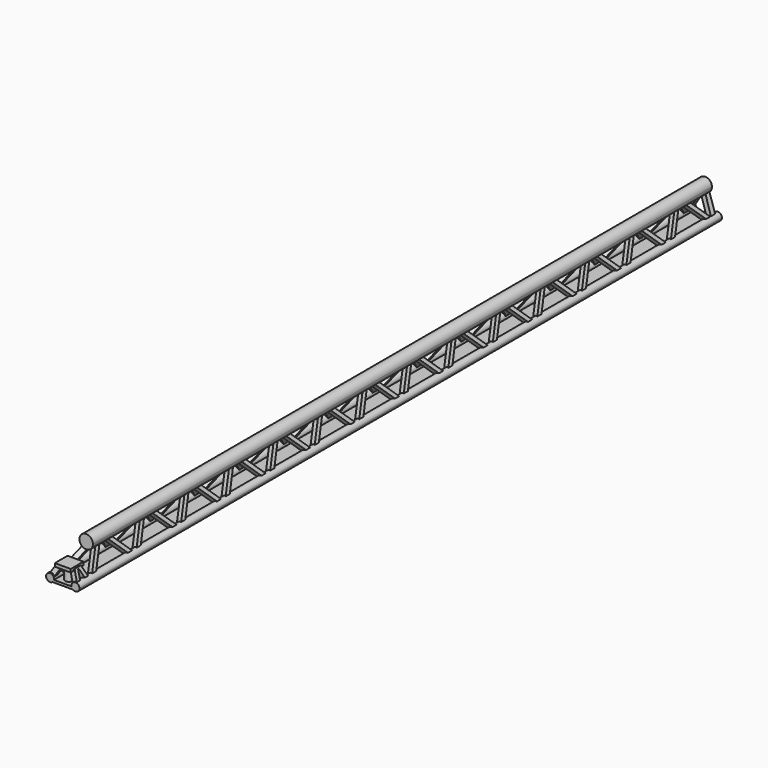
from build123d import *

# Parameters (mm, degrees)
F1_DEPTH  = 505
F4_DEPTH  = 1.5
F7_DEPTH  = 10
F8_W      = 22
F8_H      = 9.3770528809
F9_DEPTH  = 12.5
F10_R     = 2.5
F11_DEPTH = 10.5


# Not quite as in the source:
# - a feature names something its author has since deleted; it is built from what else it names


with BuildPart() as f1:
    # F0 (on Front) → F1 (new body)
    with BuildSketch(Plane.XZ):
        with BuildLine():
            ThreePointArc((2, 11.25), (3.6443449343, 12.8133930394), (4.25, 15))
            ThreePointArc((4.25, 15), (-2.1866069606, 18.6443449343), (-2, 11.25))
            Line((-2, 11.25), (0, 15))
            Line((0, 15), (2, 11.25))
        make_face()
        with BuildLine():
            Line((0, 15), (-2, 11.25))
            ThreePointArc((-2, 11.25), (0, 10.75), (2, 11.25))
            Line((2, 11.25), (0, 15))
        make_face()
    extrude(amount=F1_DEPTH)



with BuildPart() as f1b:
    # F0 (on Front) → F1, piece 2 (new body)
    with BuildSketch(Plane.XZ):
        with BuildLine():
            ThreePointArc((6.5, -2), (9.1180339887, -2.2360679775), (10.5, 0))
            ThreePointArc((10.5, 0), (7.748727595, 2.4873403825), (5.5505102572, -0.5))
            Line((5.5505102572, -0.5), (8, -0.5))
            Line((8, -0.5), (8, -2))
            Line((8, -2), (6.5, -2))
        make_face()
        with BuildLine():
            Line((8, -0.5), (5.5505102572, -0.5))
            ThreePointArc((5.5505102572, -0.5), (5.8876275643, -1.3371173071), (6.5, -2))
            Line((6.5, -2), (8, -2))
            Line((8, -2), (8, -0.5))
        make_face()
        with BuildLine():
            ThreePointArc((6.5, -2), (5.8876275643, -1.3371173071), (5.5505102572, -0.5))
            Line((5.5505102572, -0.5), (-5.5505102572, -0.5))
            ThreePointArc((-5.5505102572, -0.5), (-5.8876275643, -1.3371173071), (-6.5, -2))
            Line((-6.5, -2), (6.5, -2))
        make_face()
        with BuildLine():
            Line((-8, -0.5), (-5.5505102572, -0.5))
            ThreePointArc((-5.5505102572, -0.5), (-5.5126596175, -0.251272405), (-5.5, 0))
            ThreePointArc((-5.5, 0), (-10.2360679775, 1.1180339887), (-6.5, -2))
            Line((-6.5, -2), (-8, -2))
            Line((-8, -2), (-8, -0.5))
        make_face()
        with BuildLine():
            ThreePointArc((-6.5, -2), (-5.8876275643, -1.3371173071), (-5.5505102572, -0.5))
            Line((-5.5505102572, -0.5), (-8, -0.5))
            Line((-8, -0.5), (-8, -2))
            Line((-8, -2), (-6.5, -2))
        make_face()
    extrude(amount=F1_DEPTH)


with BuildPart() as f1_1:
    add(f1.part)

    add(f1b.part)  # F4 merges F1b
    # F3 (on face) → F4 (join, symmetric)
    with BuildSketch(Plane(origin=(-6.2283737024, 0, 3.321799308), x_dir=(0, -1, 0), z_dir=(-0.8823529412, 0, 0.4705882353))):
        Polygon((235.2386346391, 13.0811002704), (232, 13.0811002704), (246, -3.9188997296), (249.2386346391, -3.9188997296), align=None)
        Polygon((6.0693119959, -2.3306788158), (6.3806826805, -3.9188997296), (8, -3.9188997296), (22, 13.0811002704), (18.7613653609, 13.0811002704), align=None)
        Polygon((57, 13.0811002704), (53.7613653609, 13.0811002704), (39.7613653609, -3.9188997296), (43, -3.9188997296), align=None)
        Polygon((60.2386346391, 13.0811002704), (57, 13.0811002704), (71, -3.9188997296), (74.2386346391, -3.9188997296), align=None)
        Polygon((92, 13.0811002704), (88.7613653609, 13.0811002704), (74.7613653609, -3.9188997296), (78, -3.9188997296), align=None)
        Polygon((95.2386346391, 13.0811002704), (92, 13.0811002704), (106, -3.9188997296), (109.2386346391, -3.9188997296), align=None)
        Polygon((127, 13.0811002704), (123.7613653609, 13.0811002704), (109.7613653609, -3.9188997296), (113, -3.9188997296), align=None)
        Polygon((130.2386346391, 13.0811002704), (127, 13.0811002704), (141, -3.9188997296), (144.2386346391, -3.9188997296), align=None)
        Polygon((162, 13.0811002704), (158.7613653609, 13.0811002704), (144.7613653609, -3.9188997296), (148, -3.9188997296), align=None)
        Polygon((165.2386346391, 13.0811002704), (162, 13.0811002704), (176, -3.9188997296), (179.2386346391, -3.9188997296), align=None)
        Polygon((197, 13.0811002704), (193.7613653609, 13.0811002704), (179.7613653609, -3.9188997296), (183, -3.9188997296), align=None)
        Polygon((200.2386346391, 13.0811002704), (197, 13.0811002704), (211, -3.9188997296), (214.2386346391, -3.9188997296), align=None)
        Polygon((232, 13.0811002704), (228.7613653609, 13.0811002704), (214.7613653609, -3.9188997296), (218, -3.9188997296), align=None)
        Polygon((25.2386346391, 13.0811002704), (22, 13.0811002704), (36, -3.9188997296), (39.2386346391, -3.9188997296), align=None)
        Polygon((263.2386346391, 13.0811002704), (249.2386346391, -3.9188997296), (252.4772692781, -3.9188997296), (266.4772692781, 13.0811002704), align=None)
        Polygon((267, 13.0811002704), (281, -3.9188997296), (284.2386346391, -3.9188997296), (270.2386346391, 13.0811002704), align=None)
        Polygon((298.2386346391, 13.0811002704), (284.2386346391, -3.9188997296), (287.4772692781, -3.9188997296), (301.4772692781, 13.0811002704), align=None)
        Polygon((302, 13.0811002704), (316, -3.9188997296), (319.2386346391, -3.9188997296), (305.2386346391, 13.0811002704), align=None)
        Polygon((333.2386346391, 13.0811002704), (319.2386346391, -3.9188997296), (322.4772692781, -3.9188997296), (336.4772692781, 13.0811002704), align=None)
        Polygon((337, 13.0811002704), (351, -3.9188997296), (354.2386346391, -3.9188997296), (340.2386346391, 13.0811002704), align=None)
        Polygon((368.2386346391, 13.0811002704), (354.2386346391, -3.9188997296), (357.4772692781, -3.9188997296), (371.4772692781, 13.0811002704), align=None)
        Polygon((372, 13.0811002704), (386, -3.9188997296), (389.2386346391, -3.9188997296), (375.2386346391, 13.0811002704), align=None)
        Polygon((403.2386346391, 13.0811002704), (389.2386346391, -3.9188997296), (392.4772692781, -3.9188997296), (406.4772692781, 13.0811002704), align=None)
        Polygon((407, 13.0811002704), (421, -3.9188997296), (424.2386346391, -3.9188997296), (410.2386346391, 13.0811002704), align=None)
        Polygon((438.2386346391, 13.0811002704), (424.2386346391, -3.9188997296), (427.4772692781, -3.9188997296), (441.4772692781, 13.0811002704), align=None)
        Polygon((442, 13.0811002704), (456, -3.9188997296), (459.2386346391, -3.9188997296), (445.2386346391, 13.0811002704), align=None)
        Polygon((473.2386346391, 13.0811002704), (459.2386346391, -3.9188997296), (462.4772692781, -3.9188997296), (476.4772692781, 13.0811002704), align=None)
        Polygon((0, 13.0811002704), (3.0478329538, -3.9188997296), (4.7613653609, -3.9188997296), (6.0693119959, -2.3306788158), (3.0478329538, 13.0811002704), align=None)
        Polygon((477, 13.0811002704), (491, -3.9188997296), (494.2386346391, -3.9188997296), (480.2386346391, 13.0811002704), align=None)
        Polygon((497.5, 4.5811002704), (495, -3.9188997296), (497.5, -3.9188997296), (499.7058823529, 3.5811002704), (500, 3.5811002704), (500, 4.5811002704), align=None)
        Polygon((502.5, 4.5811002704), (500, 4.5811002704), (500, 3.5811002704), (500.1383992214, 3.5811002704), (500.2941176471, 3.5811002704), (502.5, -3.9188997296), (505, -3.9188997296), align=None)
    extrude(amount=F4_DEPTH, both=True)


with BuildPart() as f5_1:
    # F5: instance of F1
    add(f1_1.part.mirror(Plane.YZ))


with BuildPart() as f1_2:
    add(f1_1.part)

    add(f5_1.part)  # F7 merges F5_1
    # F6 (on face) → F7 (join)
    with BuildSketch(Plane.XZ.offset(505)):
        Polygon((-5, 7), (0, 7), (5, 7), (5, 9), (-5, 9), align=None)
    extrude(amount=-F7_DEPTH)

    # F8 (on Right) → F9 (cut, symmetric)
    with BuildSketch(Plane.YZ):
        with Locations((-497.5955486298, 14.8281380534)):
            Rectangle(F8_W, F8_H)
    extrude(amount=F9_DEPTH, both=True, mode=Mode.SUBTRACT)

    # F10 (on face) → F11 (join)
    with BuildSketch(Plane.XY.offset(9)):
        with Locations((0, -500)):
            Circle(F10_R)
    extrude(amount=-F11_DEPTH)


solid = f1_2.part
